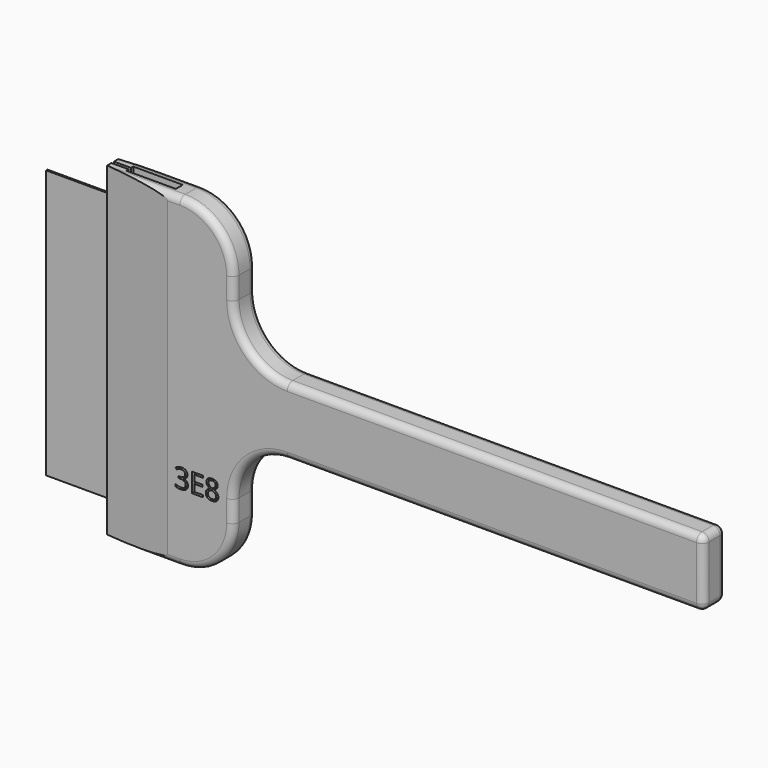
from build123d import *

# Parameters (mm, degrees)
F4_W          = 19.15
F4_H          = 39
F5_DEPTH      = 0.25
F6_W          = 7
F6_H          = 1.08
F7_DEPTH      = 39
F10_DEPTH     = 43.2
F12_DEPTH     = 4
F13_W         = 4
F13_H         = 9.75
F14_DEPTH     = 68.25
F15_R         = 7.8
F16_R         = 1
F17_TEXT_SIZE = 3.8888888889
F18_DEPTH     = 0.5


# Not quite as in the source:
# - Text() gives the source's letters only with a copy of the font that has no kerning and outlines rounded to 1/6400 em; it was checked with that copy


with BuildPart() as f5:
    # F4 (on Front) → F5 (new body)
    with BuildSketch(Plane.XZ):
        with Locations((-6.001778594, 19.5)):
            Rectangle(F4_W, F4_H)
    extrude(amount=F5_DEPTH)

    # F6 (on face) → F7 (join, through all)
    with BuildSketch(Plane(origin=(0, 0, 0), x_dir=(1, 0, 0), z_dir=(0, 0, -1))):
        with Locations((0.073221406, 0.125)):
            Rectangle(F6_W, F6_H)
    extrude(amount=-F7_DEPTH)


with BuildPart() as f10:
    # F9 (on offset) → F10 (new body)
    with BuildSketch(Plane(origin=(0, 0, -0.1), x_dir=(1, 0, 0), z_dir=(0, 0, -1))):
        Polygon((3.673221406, -0.515), (-3.526778594, -0.515), (-3.526778594, -0.1), (-6.001778594, -0.1), (-6.001778594, -0.875), (3.573221406, -1.875), (13.148221406, -1.875), (13.148221406, 2.125), (3.573221406, 2.125), (-6.001778594, 1.125), (-6.001778594, 0.35), (-3.526778594, 0.35), (-3.526778594, 0.765), (3.673221406, 0.765), align=None)
    extrude(amount=-F10_DEPTH)

    # F11 (on face) → F12 (join)
    with BuildSketch(Plane(origin=(0, 0, -0.1), x_dir=(1, 0, 0), z_dir=(0, 0, -1))):
        Polygon((-6.001778594, 0.35), (-6.001778594, -0.1), (-6.001778594, -0.875), (3.573221406, -1.875), (13.148221406, -1.875), (13.148221406, 2.125), (3.573221406, 2.125), (-6.001778594, 1.125), align=None)
    extrude(amount=F12_DEPTH)

    # F13 (on face) → F14 (join)
    with BuildSketch(Plane.YZ.offset(13.148221406)):
        with Locations((-0.125, 19.5)):
            Rectangle(F13_W, F13_H)
    extrude(amount=F14_DEPTH)

    # F15
    f15_edges = [f10.edges().sort_by_distance(p)[0] for p in [
        (13.148221, -0.125, 24.375),
        (13.148221, -0.125, 43.1),
        (13.148221, -0.125, -4.1),
        (13.148221, -0.125, 14.625),
    ]]
    fillet(f15_edges, radius=F15_R)

    # F16
    f16_edges = [f10.edges().sort_by_distance(p)[0] for p in [
        (81.398221, -0.125, 24.375),
        (81.398221, -2.125, 19.5),
        (81.398221, -0.125, 14.625),
        (81.398221, 1.875, 19.5),
        (51.173221, -2.125, 24.375),
        (51.173221, 1.875, 24.375),
        (51.173221, -2.125, 14.625),
        (51.173221, 1.875, 14.625),
    ]]
    fillet(f16_edges, radius=F16_R)

    # F17 (on face) → F18 (cut)
    with BuildSketch(Plane.XZ.offset(2.125)):
        with Locations((4.5347195315, 5.858336944)):
            Text('3E8', F17_TEXT_SIZE, font='Open Sans', text_align=(TextAlign.LEFT, TextAlign.BOTTOM))
    extrude(amount=-F18_DEPTH, mode=Mode.SUBTRACT)


solid = Compound([f5.part, f10.part])
